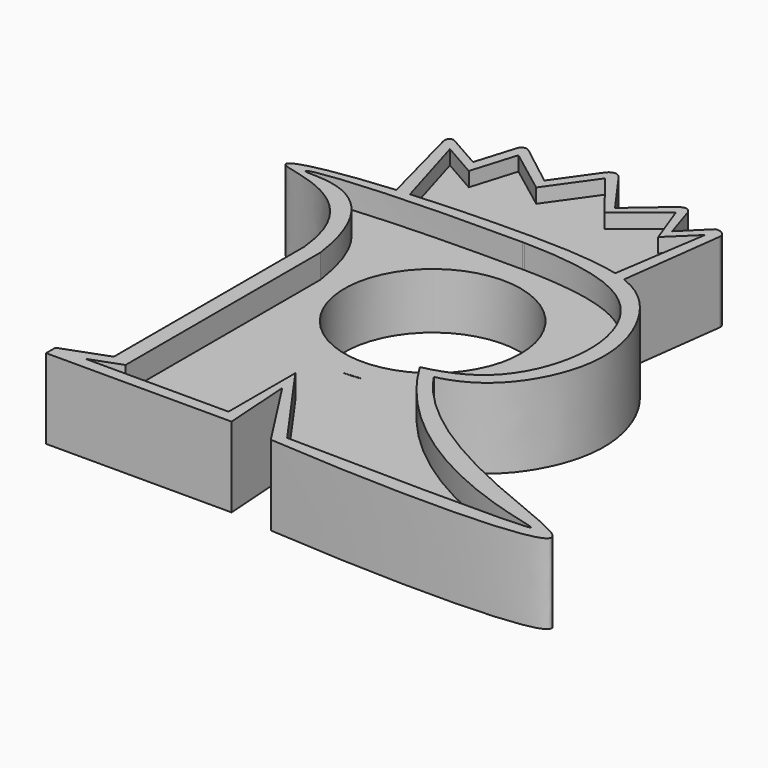
from build123d import *

# Parameters (mm, degrees)
F1_DEPTH = 10
F0_R     = 11.025
F2_DEPTH = 7
F3_DEPTH = 8.2


with BuildPart() as f1:
    # F0 (on Top) → F1 (new body)
    with BuildSketch(Plane.XY):
        with BuildLine():
            Line((-19.3000361323, 25.617852807), (-16.5027223659, 14.9471961935))
            add(Edge.make_bspline(
                [(-16.5027223659, 14.9471961935), (-15.9821834932, 14.9908863575), (-15.4454033317, 15.0328594986), (-14.8925539408, 15.0729105388)],
                knots=[0.8146444204, 0.8146444204, 0.8146444204, 0.8146444204, 0.8366556125, 0.8366556125, 0.8366556125, 0.8366556125], degree=3))
            Line((-14.8925539408, 15.0729105388), (-17.8214006024, 24.9819634817))
            Line((-17.8214006024, 24.9819634817), (-13.4857874364, 22.5029587746))
            Line((-13.4857874364, 22.5029587746), (-11.7759136483, 28.1340777874))
            Line((-11.7759136483, 28.1340777874), (-6.1606834643, 23.8938014954))
            Line((-6.1606834643, 23.8938014954), (-2.1075964905, 29.6155139804))
            Line((-2.1075964905, 29.6155139804), (2.369817812, 23.8938014954))
            Line((2.369817812, 23.8938014954), (7.7946316451, 28.2900184393))
            Line((7.7946316451, 28.2900184393), (9.6949217841, 23.1520179659))
            Line((9.6949217841, 23.1520179659), (12.9975004857, 26.3469954851))
            Line((12.9975004857, 26.3469954851), (11.199255367, 14.5383238121))
            add(Edge.make_bspline(
                [(11.199255367, 14.5383238121), (11.7299576144, 14.3959369713), (12.2254180774, 14.2360425799), (12.6910973587, 14.05701797)],
                knots=[0.1587326419, 0.1587326419, 0.1587326419, 0.1587326419, 0.1906610807, 0.1906610807, 0.1906610807, 0.1906610807], degree=3))
            Line((12.6910973587, 14.05701797), (14.3530135974, 27.0172487944))
            add(Edge.make_bspline(
                [(13.0104408682, 27.9140680165), (13.5631300509, 28.1455442309), (14.3618108705, 27.6210475713), (14.3530135974, 27.0172487944)],
                knots=[0, 0, 0, 0, 1.6145545052, 1.6145545052, 1.6145545052, 1.6145545052], degree=3))
            Line((13.0104408682, 27.9140680165), (10.0033283234, 24.9562524259))
            Line((10.0033283234, 24.9562524259), (8.6801284924, 29.0636848658))
            add(Edge.make_bspline(
                [(8.6801284924, 29.0636848658), (8.282721974, 29.7467447817), (7.8180013224, 29.7191031277), (7.1373213177, 29.2566530406)],
                knots=[0, 0, 0, 0, 1.5548281882, 1.5548281882, 1.5548281882, 1.5548281882], degree=3))
            Line((7.1373213177, 29.2566530406), (2.5603291579, 25.3146197647))
            Line((2.5603291579, 25.3146197647), (-1.2397119331, 30.6349862367))
            add(Edge.make_bspline(
                [(-2.8427368961, 30.6349862367), (-2.3610445205, 31.2117636204), (-1.6856613802, 31.2255471945), (-1.2397119331, 30.6349862367)],
                knots=[0, 0, 0, 0, 1.603024963, 1.603024963, 1.603024963, 1.603024963], degree=3))
            Line((-2.8427368961, 30.6349862367), (-6.4539699815, 25.5351532251))
            Line((-6.4539699815, 25.5351532251), (-11.6916364059, 29.5874532312))
            add(Edge.make_bspline(
                [(-12.7943027765, 29.3117854744), (-12.6205328852, 29.7315195203), (-12.1682910249, 29.876427725), (-11.6916364059, 29.5874532312)],
                knots=[0, 0, 0, 0, 1.1366027613, 1.1366027613, 1.1366027613, 1.1366027613], degree=3))
            Line((-12.7943027765, 29.3117854744), (-14.3380360678, 24.239519611))
            Line((-14.3380360678, 24.239519611), (-18.7211353332, 26.7205201089))
            add(Edge.make_bspline(
                [(-18.7211353332, 26.7205201089), (-19.4361973554, 26.7992690206), (-19.4751825184, 26.2437313795), (-19.3000361323, 25.617852807)],
                knots=[0, 0, 0, 0, 1.2453920322, 1.2453920322, 1.2453920322, 1.2453920322], degree=3))
        make_face()
        with BuildLine():
            add(Edge.make_bspline(
                [(-16.0178430378, 0), (-17.0891042799, 11.2457247451), (-34.3895874626, 11.4951487861), (-25.4101731911, 14.199570976), (-16.5027223659, 14.9471961935)],
                knots=[0, 0, 0, 0, 0.4379893378, 0.8146444204, 0.8146444204, 0.8146444204, 0.8146444204], degree=3))
            Line((-16.0178430378, 0), (-16.0178430378, -29.8405252397))
            Line((-16.0178430378, -29.8405252397), (-21.6572081245, -31.9249667227))
            Line((-21.6572081245, -31.9249667227), (-21.6572081245, -33.3810336888))
            Line((-21.6572081245, -33.3810336888), (1.5535618877, -33.3810336888))
            Line((1.5535618877, -33.3810336888), (0.9634781745, -24.7264597565))
            Line((0.9634781745, -24.7264597565), (6.929886993, -33.9711159468))
            add(Edge.make_bspline(
                [(6.929886993, -33.9711159468), (24.8493433086, -35.2838962809), (60.3720002804, -34.8670480548), (19.1815471681, -25.9585702534), (11.0604790971, -13.6459805071)],
                knots=[0, 0, 0, 0, 0.4949574997, 1, 1, 1, 1], degree=3))
            add(Edge.make_bspline(
                [(12.6910973587, 14.05701797), (14.3809471326, 13.4073762346), (18.5460833461, 10.5137101685), (23.2371850237, 0.0289954641), (17.8748979072, -11.1493005541), (12.8722470254, -13.2691906765), (11.0604790971, -13.6459805071)],
                knots=[0.1906610807, 0.1906610807, 0.1906610807, 0.1906610807, 0.3065225054, 0.5625365171, 0.8107732693, 1, 1, 1, 1], degree=3))
            add(Edge.make_bspline(
                [(11.199255367, 14.5383238121), (11.7299576144, 14.3959369713), (12.2254180774, 14.2360425799), (12.6910973587, 14.05701797)],
                knots=[0.1587326419, 0.1587326419, 0.1587326419, 0.1587326419, 0.1906610807, 0.1906610807, 0.1906610807, 0.1906610807], degree=3))
            add(Edge.make_bspline(
                [(0, 15.5631974339), (5.0514355202, 15.5213642545), (8.5608623501, 15.246201814), (11.199255367, 14.5383238121)],
                knots=[0, 0, 0, 0, 0.1587326419, 0.1587326419, 0.1587326419, 0.1587326419], degree=3))
            add(Edge.make_bspline(
                [(-14.8925539408, 15.0729105388), (-10.7898754349, 15.3701280895), (-5.8022517829, 15.5614940305), (0, 15.5631974339)],
                knots=[0.8366556125, 0.8366556125, 0.8366556125, 0.8366556125, 1, 1, 1, 1], degree=3))
            add(Edge.make_bspline(
                [(-16.5027223659, 14.9471961935), (-15.9821834932, 14.9908863575), (-15.4454033317, 15.0328594986), (-14.8925539408, 15.0729105388)],
                knots=[0.8146444204, 0.8146444204, 0.8146444204, 0.8146444204, 0.8366556125, 0.8366556125, 0.8366556125, 0.8366556125], degree=3))
        make_face()
        with BuildLine():
            add(Edge.make_bspline(
                [(0, 14.025), (-22.2927219479, 14.1532437558), (-32.5429377718, 11.2364486318), (-15.8938150439, 13.1059148162), (-14.025, 0)],
                knots=[0, 0, 0, 0, 0.5515868686, 1, 1, 1, 1], degree=3))
            ThreePointArc((0, 14.025), (0.1451418598, 14.0242489582), (0.2902681747, 14.0219959131))
            add(Edge.make_bspline(
                [(0.2902681747, 14.0219959131), (9.2486399688, 13.9105710304), (17.0995105355, 10.759716712), (20.385285187, 0.0139246379), (16.8992797962, -9.7633800937), (11.6691263972, -12.2065090216), (8.7014966008, -12.8828223231)],
                knots=[0.0030566307, 0.0030566307, 0.0030566307, 0.0030566307, 0.2875779073, 0.4994840668, 0.7217267051, 0.8772385131, 0.8772385131, 0.8772385131, 0.8772385131], degree=3))
            add(Edge.make_bspline(
                [(7.9412147987, -32.6805368676), (13.8764368589, -32.813362548), (60.0064221878, -33.4995761154), (19.4618183039, -30.7597754392), (8.7014966151, -12.8828223083)],
                knots=[0, 0, 0, 0, 0.4752172088, 0.9876392002, 0.9876392002, 0.9876392002, 0.9876392002], degree=3))
            Line((7.9412147987, -32.6805368676), (0, -21.472029388))
            Line((0, -21.472029388), (0, -31.9249667227))
            Line((0, -31.9249667227), (-17.9133024067, -31.9249667227))
            Line((-17.9133024067, -31.9249667227), (-14.025, -30.4877590388))
            Line((-14.025, -30.4877590388), (-14.025, 0))
        make_face(mode=Mode.SUBTRACT)
    extrude(amount=F1_DEPTH)

    # F0 (on Top) → F2 (join)
    with BuildSketch(Plane.XY):
        with BuildLine():
            add(Edge.make_bspline(
                [(-16.0178430378, 0), (-17.0891042799, 11.2457247451), (-34.3895874626, 11.4951487861), (-25.4101731911, 14.199570976), (-16.5027223659, 14.9471961935)],
                knots=[0, 0, 0, 0, 0.4379893378, 0.8146444204, 0.8146444204, 0.8146444204, 0.8146444204], degree=3))
            Line((-16.0178430378, 0), (-16.0178430378, -29.8405252397))
            Line((-16.0178430378, -29.8405252397), (-21.6572081245, -31.9249667227))
            Line((-21.6572081245, -31.9249667227), (-21.6572081245, -33.3810336888))
            Line((-21.6572081245, -33.3810336888), (1.5535618877, -33.3810336888))
            Line((1.5535618877, -33.3810336888), (0.9634781745, -24.7264597565))
            Line((0.9634781745, -24.7264597565), (6.929886993, -33.9711159468))
            add(Edge.make_bspline(
                [(6.929886993, -33.9711159468), (24.8493433086, -35.2838962809), (60.3720002804, -34.8670480548), (19.1815471681, -25.9585702534), (11.0604790971, -13.6459805071)],
                knots=[0, 0, 0, 0, 0.4949574997, 1, 1, 1, 1], degree=3))
            add(Edge.make_bspline(
                [(12.6910973587, 14.05701797), (14.3809471326, 13.4073762346), (18.5460833461, 10.5137101685), (23.2371850237, 0.0289954641), (17.8748979072, -11.1493005541), (12.8722470254, -13.2691906765), (11.0604790971, -13.6459805071)],
                knots=[0.1906610807, 0.1906610807, 0.1906610807, 0.1906610807, 0.3065225054, 0.5625365171, 0.8107732693, 1, 1, 1, 1], degree=3))
            add(Edge.make_bspline(
                [(11.199255367, 14.5383238121), (11.7299576144, 14.3959369713), (12.2254180774, 14.2360425799), (12.6910973587, 14.05701797)],
                knots=[0.1587326419, 0.1587326419, 0.1587326419, 0.1587326419, 0.1906610807, 0.1906610807, 0.1906610807, 0.1906610807], degree=3))
            add(Edge.make_bspline(
                [(0, 15.5631974339), (5.0514355202, 15.5213642545), (8.5608623501, 15.246201814), (11.199255367, 14.5383238121)],
                knots=[0, 0, 0, 0, 0.1587326419, 0.1587326419, 0.1587326419, 0.1587326419], degree=3))
            add(Edge.make_bspline(
                [(-14.8925539408, 15.0729105388), (-10.7898754349, 15.3701280895), (-5.8022517829, 15.5614940305), (0, 15.5631974339)],
                knots=[0.8366556125, 0.8366556125, 0.8366556125, 0.8366556125, 1, 1, 1, 1], degree=3))
            add(Edge.make_bspline(
                [(-16.5027223659, 14.9471961935), (-15.9821834932, 14.9908863575), (-15.4454033317, 15.0328594986), (-14.8925539408, 15.0729105388)],
                knots=[0.8146444204, 0.8146444204, 0.8146444204, 0.8146444204, 0.8366556125, 0.8366556125, 0.8366556125, 0.8366556125], degree=3))
        make_face()
        with BuildLine():
            add(Edge.make_bspline(
                [(0, 14.025), (-22.2927219479, 14.1532437558), (-32.5429377718, 11.2364486318), (-15.8938150439, 13.1059148162), (-14.025, 0)],
                knots=[0, 0, 0, 0, 0.5515868686, 1, 1, 1, 1], degree=3))
            ThreePointArc((0, 14.025), (0.1451418598, 14.0242489582), (0.2902681747, 14.0219959131))
            add(Edge.make_bspline(
                [(0.2902681747, 14.0219959131), (9.2486399688, 13.9105710304), (17.0995105355, 10.759716712), (20.385285187, 0.0139246379), (16.8992797962, -9.7633800937), (11.6691263972, -12.2065090216), (8.7014966008, -12.8828223231)],
                knots=[0.0030566307, 0.0030566307, 0.0030566307, 0.0030566307, 0.2875779073, 0.4994840668, 0.7217267051, 0.8772385131, 0.8772385131, 0.8772385131, 0.8772385131], degree=3))
            add(Edge.make_bspline(
                [(7.9412147987, -32.6805368676), (13.8764368589, -32.813362548), (60.0064221878, -33.4995761154), (19.4618183039, -30.7597754392), (8.7014966151, -12.8828223083)],
                knots=[0, 0, 0, 0, 0.4752172088, 0.9876392002, 0.9876392002, 0.9876392002, 0.9876392002], degree=3))
            Line((7.9412147987, -32.6805368676), (0, -21.472029388))
            Line((0, -21.472029388), (0, -31.9249667227))
            Line((0, -31.9249667227), (-17.9133024067, -31.9249667227))
            Line((-17.9133024067, -31.9249667227), (-14.025, -30.4877590388))
            Line((-14.025, -30.4877590388), (-14.025, 0))
        make_face(mode=Mode.SUBTRACT)
        with BuildLine():
            ThreePointArc((0, -14.025), (-9.9171726061, -9.9171726061), (-14.025, 0))
            Line((-14.025, 0), (-14.025, -30.4877590388))
            Line((-14.025, -30.4877590388), (-17.9133024067, -31.9249667227))
            Line((-17.9133024067, -31.9249667227), (0, -31.9249667227))
            Line((0, -31.9249667227), (0, -21.472029388))
            Line((0, -21.472029388), (7.9412147987, -32.6805368676))
            add(Edge.make_bspline(
                [(7.9412147987, -32.6805368676), (13.8764368589, -32.813362548), (60.0064221878, -33.4995761154), (19.4618183039, -30.7597754392), (8.7014966151, -12.8828223083)],
                knots=[0, 0, 0, 0, 0.4752172088, 0.9876392002, 0.9876392002, 0.9876392002, 0.9876392002], degree=3))
            add(Edge.make_bspline(
                [(8.7014966008, -12.8828223231), (6.9291756993, -13.2867285657), (4.8663444244, -13.5731266075), (2.4476929742, -13.8097582927)],
                knots=[0.8772385131, 0.8772385131, 0.8772385131, 0.8772385131, 0.9701129101, 0.9701129101, 0.9701129101, 0.9701129101], degree=3))
            ThreePointArc((2.4476929742, -13.8097582927), (1.2285692785, -13.9710859466), (0, -14.025))
        make_face()
        with BuildLine():
            add(Edge.make_bspline(
                [(0, 14.025), (0.0972728272, 14.0241944405), (0.1940278004, 14.0231929579), (0.2902681747, 14.0219959131)],
                knots=[0, 0, 0, 0, 0.0030566307, 0.0030566307, 0.0030566307, 0.0030566307], degree=3))
            ThreePointArc((0, 14.025), (-9.9171726061, 9.9171726061), (-14.025, 0))
            ThreePointArc((-14.025, 0), (-9.9171726061, -9.9171726061), (0, -14.025))
            add(Edge.make_bspline(
                [(2.4476929742, -13.8097582927), (1.6693680994, -13.8859066467), (0.8541959122, -13.9569013961), (0, -14.025)],
                knots=[0.9701129101, 0.9701129101, 0.9701129101, 0.9701129101, 1, 1, 1, 1], degree=3))
            ThreePointArc((2.4476929742, -13.8097582927), (5.3148380237, -12.9789491786), (7.9412147987, -11.5601787409))
            ThreePointArc((7.9412147987, -11.5601787409), (12.4112078895, -6.5316570428), (14.025, 0))
            ThreePointArc((14.025, 0), (10.0192723326, 9.8140107461), (0.2902681747, 14.0219959131))
        make_face()
        Circle(F0_R, mode=Mode.SUBTRACT)
        with BuildLine():
            add(Edge.make_bspline(
                [(0.2902681747, 14.0219959131), (9.2486399688, 13.9105710304), (17.0995105355, 10.759716712), (20.385285187, 0.0139246379), (16.8992797962, -9.7633800937), (11.6691263972, -12.2065090216), (8.7014966008, -12.8828223231)],
                knots=[0.0030566307, 0.0030566307, 0.0030566307, 0.0030566307, 0.2875779073, 0.4994840668, 0.7217267051, 0.8772385131, 0.8772385131, 0.8772385131, 0.8772385131], degree=3))
            ThreePointArc((0.2902681747, 14.0219959131), (10.0192723326, 9.8140107461), (14.025, 0))
            ThreePointArc((14.025, 0), (12.4112078895, -6.5316570428), (7.9412147987, -11.5601787409))
            add(Edge.make_bspline(
                [(8.7014966151, -12.8828223083), (8.4419328487, -12.4515889846), (8.1883483332, -12.0107804723), (7.9412147987, -11.5601787409)],
                knots=[0.9876392002, 0.9876392002, 0.9876392002, 0.9876392002, 1, 1, 1, 1], degree=3))
        make_face()
        with BuildLine():
            ThreePointArc((-14.025, 0), (-9.9171726061, 9.9171726061), (0, 14.025))
            add(Edge.make_bspline(
                [(0, 14.025), (-22.2927219479, 14.1532437558), (-32.5429377718, 11.2364486318), (-15.8938150439, 13.1059148162), (-14.025, 0)],
                knots=[0, 0, 0, 0, 0.5515868686, 1, 1, 1, 1], degree=3))
        make_face()
        with BuildLine():
            add(Edge.make_bspline(
                [(8.7014966008, -12.8828223231), (6.9291756993, -13.2867285657), (4.8663444244, -13.5731266075), (2.4476929742, -13.8097582927)],
                knots=[0.8772385131, 0.8772385131, 0.8772385131, 0.8772385131, 0.9701129101, 0.9701129101, 0.9701129101, 0.9701129101], degree=3))
            add(Edge.make_bspline(
                [(8.7014966151, -12.8828223083), (8.4419328487, -12.4515889846), (8.1883483332, -12.0107804723), (7.9412147987, -11.5601787409)],
                knots=[0.9876392002, 0.9876392002, 0.9876392002, 0.9876392002, 1, 1, 1, 1], degree=3))
            ThreePointArc((7.9412147987, -11.5601787409), (5.3148380237, -12.9789491786), (2.4476929742, -13.8097582927))
        make_face()
        with BuildLine():
            ThreePointArc((0.2902681747, 14.0219959131), (0.1451418598, 14.0242489582), (0, 14.025))
            add(Edge.make_bspline(
                [(0, 14.025), (0.0972728272, 14.0241944405), (0.1940278004, 14.0231929579), (0.2902681747, 14.0219959131)],
                knots=[0, 0, 0, 0, 0.0030566307, 0.0030566307, 0.0030566307, 0.0030566307], degree=3))
        make_face()
    extrude(amount=F2_DEPTH)

    # F0 (on Top) → F3 (join)
    with BuildSketch(Plane.XY):
        with BuildLine():
            Line((-17.8214006024, 24.9819634817), (-14.8925539408, 15.0729105388))
            add(Edge.make_bspline(
                [(-14.8925539408, 15.0729105388), (-10.7898754349, 15.3701280895), (-5.8022517829, 15.5614940305), (0, 15.5631974339)],
                knots=[0.8366556125, 0.8366556125, 0.8366556125, 0.8366556125, 1, 1, 1, 1], degree=3))
            add(Edge.make_bspline(
                [(0, 15.5631974339), (5.0514355202, 15.5213642545), (8.5608623501, 15.246201814), (11.199255367, 14.5383238121)],
                knots=[0, 0, 0, 0, 0.1587326419, 0.1587326419, 0.1587326419, 0.1587326419], degree=3))
            Line((11.199255367, 14.5383238121), (12.9975004857, 26.3469954851))
            Line((12.9975004857, 26.3469954851), (9.6949217841, 23.1520179659))
            Line((9.6949217841, 23.1520179659), (7.7946316451, 28.2900184393))
            Line((7.7946316451, 28.2900184393), (2.369817812, 23.8938014954))
            Line((2.369817812, 23.8938014954), (-2.1075964905, 29.6155139804))
            Line((-2.1075964905, 29.6155139804), (-6.1606834643, 23.8938014954))
            Line((-6.1606834643, 23.8938014954), (-11.7759136483, 28.1340777874))
            Line((-11.7759136483, 28.1340777874), (-13.4857874364, 22.5029587746))
            Line((-13.4857874364, 22.5029587746), (-17.8214006024, 24.9819634817))
        make_face()
    extrude(amount=F3_DEPTH)


solid = f1.part
